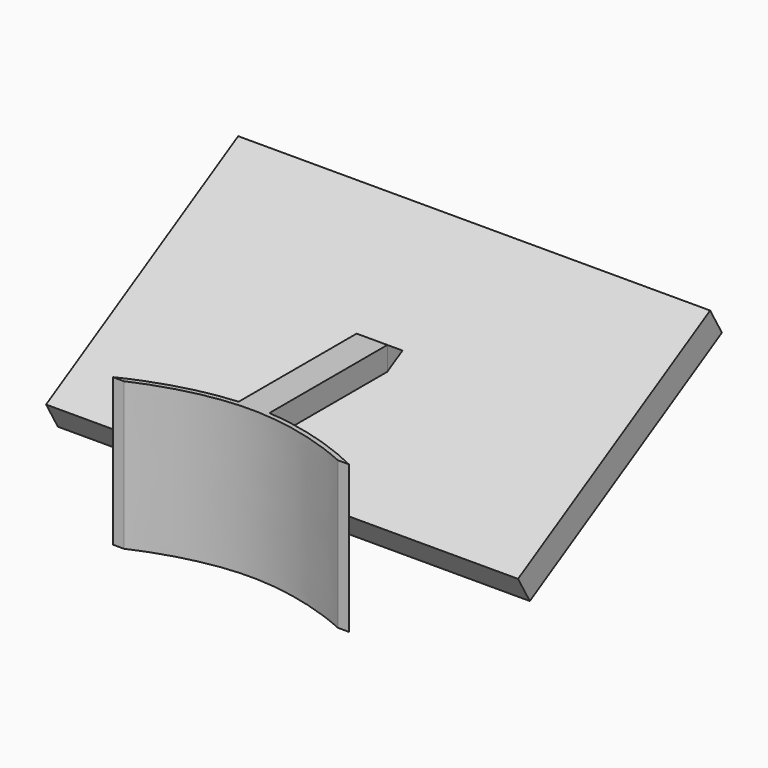
from build123d import *

# Parameters (mm, degrees)
F1_DEPTH  = 125
F3_DEPTH  = 20
F5_DEPTH  = 187
F7_DEPTH  = 213
F8_W      = 370
F8_H      = 205
F9_DEPTH  = 3
F10_W     = 15
F10_H     = 6
F10_W_2   = 20
F11_DEPTH = 3
F13_DEPTH = 26


# Not quite as in the source:
# - ends of sketch curves that miss each other by under 0.0002 mm in the source are joined
# - the dataset's text gives a spline's control points without its knots; the knots are read off the source's solid


with BuildPart() as f1:
    # F0 (on Top) → F1 (new body)
    with BuildSketch(Plane.XY):
        with BuildLine():
            Line((0, -29), (0, -25))
            add(Edge.make_bspline(
                [(-100, -50), (-75, -37.5), (-37.5, -25), (0, -25)],
                knots=[0, 0, 0, 0, 0.5, 0.5, 0.5, 0.5], degree=3))
            Line((-100, -50), (-90.6944093778, -50))
            add(Edge.make_bspline(
                [(-90.6944093778, -50), (-86.5987449165, -48.1438234757), (-75.0967566586, -43.3127738232), (-58.0512990615, -37.6313364396), (-40.7635580102, -33.4057717813), (-27.3839101667, -30.9603889359), (-16.0168642352, -29.6446162761), (-6.8676046006, -29.0953479652), (-2.2892015335, -29), (0, -29)],
                knots=[0.0487321749, 0.0487321749, 0.0487321749, 0.0487321749, 0.125, 0.25, 0.3125, 0.375, 0.4375, 0.46875, 0.5, 0.5, 0.5, 0.5], degree=3))
        make_face()
        with BuildLine():
            add(Edge.make_bspline(
                [(0, -25), (37.5, -25), (75, -37.5), (100, -50)],
                knots=[0.5, 0.5, 0.5, 0.5, 1, 1, 1, 1], degree=3))
            Line((0, -25), (0, -29))
            add(Edge.make_bspline(
                [(0, -29), (2.2892015335, -29), (6.8676046006, -29.0953479652), (16.0168642352, -29.6446162761), (27.3839101667, -30.9603889359), (40.7635580102, -33.4057717813), (58.0512990615, -37.6313364396), (75.0967566586, -43.3127738232), (86.5987449165, -48.1438234757), (90.6944093778, -50.0000690471)],
                knots=[0.5, 0.5, 0.5, 0.5, 0.53125, 0.5625, 0.625, 0.6875, 0.75, 0.875, 0.9512678251, 0.9512678251, 0.9512678251, 0.9512678251], degree=3))
            Line((90.6944093778, -50.0000690471), (100, -50))
        make_face()
    extrude(amount=F1_DEPTH)

    # F2 (on face) → F3 (join)
    with BuildSketch(Plane.XY.offset(125)):
        with BuildLine():
            Line((-13, 0), (0, 0))
            Line((0, 0), (0, -25))
            add(Edge.make_bspline(
                [(13.0421580745, -25.4859430767), (8.7078145989, -25.1685023002), (4.3539072994, -25), (0, -25)],
                knots=[0.9419479027, 0.9419479027, 0.9419479027, 0.9419479027, 1, 1, 1, 1], degree=3))
            Line((13.0421580745, -25.4859430767), (13.0421580745, 0.5756272936))
            Line((13.0421580745, 0.5756272936), (13.0421580745, 99.5140569233))
            Line((13.0421580745, 99.5140569233), (-13, 99.5140569233))
            Line((-13, 99.5140569233), (-13, 0))
        make_face()
        with BuildLine():
            Line((0, -25), (0, 0))
            Line((0, 0), (-13, 0))
            Line((-13, 0), (-13, -25.4828602254))
            add(Edge.make_bspline(
                [(0, -25), (-4.339791385, -25), (-8.67958277, -25.1674114601), (-13, -25.4828602254)],
                knots=[1, 1, 1, 1, 1.0578638851, 1.0578638851, 1.0578638851, 1.0578638851], degree=3))
        make_face()
    extrude(amount=-F3_DEPTH)


with BuildPart() as f5:
    # F4 (on face) → F5 (new body)
    with BuildSketch(Plane(origin=(-13, 0, 0), x_dir=(0, -1, 0), z_dir=(-1, 0, 0))):
        Polygon((-4.251262507, 50), (-99.5140569233, 105), (-207.7672323963, 167.5), (-220.2672323963, 145.8493649054), (-16.751262507, 28.3493649054), align=None)
    extrude(amount=F5_DEPTH)

    # F6 (on face) → F7 (join)
    with BuildSketch(Plane.YZ.offset(-13)):
        Polygon((220.2672323963, 145.8493649054), (207.7672323963, 167.5), (4.251262507, 50), (16.751262507, 28.3493649054), align=None)
    extrude(amount=F7_DEPTH)

    # F8 (on face) → F9 (cut)
    with BuildSketch(Plane(origin=(0, -8.0878194679, 14.0085142408), x_dir=(1, 0, 0), z_dir=(0, 0.5, -0.8660254038))):
        with Locations((0, -146.1817013292)):
            Rectangle(F8_W, F8_H)
    extrude(amount=-F9_DEPTH, mode=Mode.SUBTRACT)

    # F10 (on face) → F11 (join)
    with BuildSketch(Plane(origin=(0, -8.0878194679, 14.0085142408), x_dir=(1, 0, 0), z_dir=(0, 0.5, -0.8660254038))):
        with Locations((-62.5, -34.6817013292)):
            Rectangle(F10_W, F10_H)
        with Locations((-84.5, -34.6817013292)):
            Rectangle(F10_W, F10_H)
        with Locations((-106.5, -34.6817013292)):
            Rectangle(F10_W, F10_H)
        with Locations((-128.5, -34.6817013292)):
            Rectangle(F10_W, F10_H)
        with Locations((-150.5, -34.6817013292)):
            Rectangle(F10_W, F10_H)
        with Locations((-175, -34.6817013292)):
            Rectangle(F10_W_2, F10_H)
    extrude(amount=F11_DEPTH)


with BuildPart() as f13:
    # F12 (on face) → F13 (new body)
    with BuildSketch(Plane(origin=(-13, 0, 0), x_dir=(0, -1, 0), z_dir=(-1, 0, 0))):
        Polygon((-99.5140569233, 105), (-99.5140569233, 125), (-115.7948323081, 114.1461497434), align=None)
    extrude(amount=-F13_DEPTH)


solid = Compound([f1.part, f5.part, f13.part])
